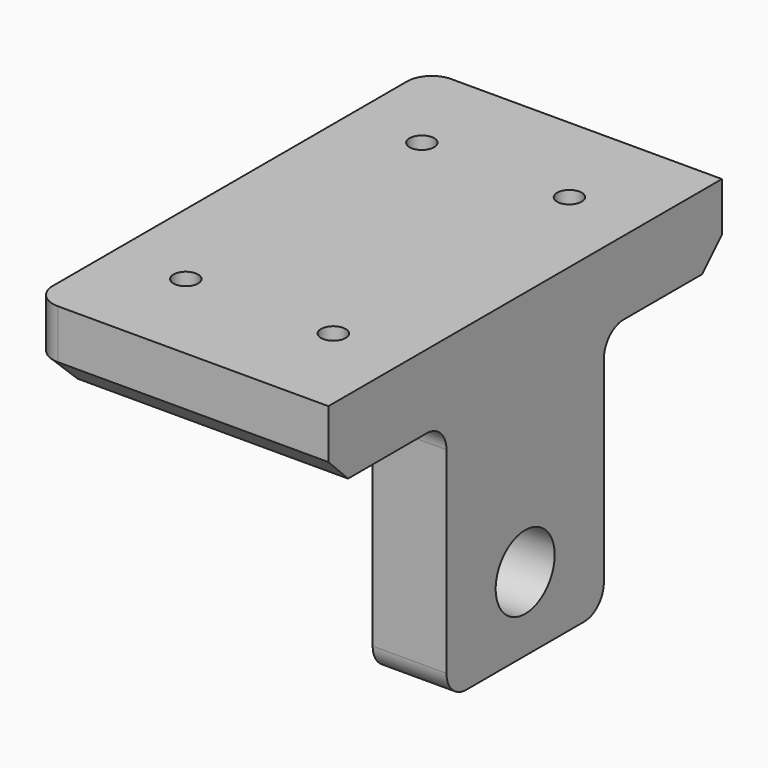
from build123d import *

# Parameters (mm, degrees)
F1_DEPTH  = 15
F2_W      = 40
F2_H      = 50
F3_DEPTH  = 15
F5_R      = 5
F6_SIZE   = 4.99999
F8_DEPTH  = 25
F9_R      = 2.5
F10_DEPTH = 25


# Not quite as in the source:
# - a fillet or chamfer is up to 0.001 mm smaller than in the source, because OpenCascade refuses the exact size


with BuildPart() as f1:
    # F0 (on Top) → F1 (new body)
    with BuildSketch(Plane.XY):
        with BuildLine():
            Line((30, 50), (-25, 50))
            ThreePointArc((-25, 50), (-28.5355339059, 48.5355339059), (-30, 45))
            Line((-30, 45), (-30, -45))
            ThreePointArc((-30, -45), (-28.5355339059, -48.5355339059), (-25, -50))
            Line((-25, -50), (30, -50))
            Line((30, -50), (30, 50))
        make_face()
    extrude(amount=F1_DEPTH)


with BuildPart() as f3:
    # F2 (on face) → F3 (new body)
    with BuildSketch(Plane.YZ.offset(30)):
        with Locations((0, -25)):
            Rectangle(F2_W, F2_H)
    extrude(amount=-F3_DEPTH)

    # F4: union F1
    add(f1.part)

    # F5
    f5_edges = [f3.edges().sort_by_distance(p)[0] for p in [
        (15, 0, 0),
        (22.5, 20, -50),
        (22.5, -20, -50),
        (22.5, 20, 0),
        (22.5, -20, 0),
    ]]
    fillet(f5_edges, radius=F5_R)

    # F6 (size 5 in the source; OpenCascade refuses exactly that, so slightly less here)
    f6_edges = [f3.edges().sort_by_distance(p)[0] for p in [
        (-30, 0, 0),
        (2.5, 50, 0),
        (2.5, -50, 0),
    ]]
    chamfer(f6_edges, length=F6_SIZE)

    # F7 (on face) → F8 (cut)
    with BuildSketch(Plane(origin=(15, 0, 0), x_dir=(0, -1, 0), z_dir=(-1, 0, 0))):
        with BuildLine():
            Line((0, -27.5), (0, -42.5))
            ThreePointArc((0, -42.5), (5.3033008589, -40.3033008589), (7.5, -35))
            ThreePointArc((7.5, -35), (5.3033008589, -29.6966991411), (0, -27.5))
        make_face()
        with BuildLine():
            ThreePointArc((0, -27.5), (-7.5, -35), (0, -42.5))
            Line((0, -42.5), (0, -27.5))
        make_face()
    extrude(amount=-F8_DEPTH, mode=Mode.SUBTRACT)

    # F9 (on face) → F10 (cut)
    with BuildSketch(Plane.XY.offset(15)):
        with Locations((-15, -30)):
            Circle(F9_R)
        with Locations((-15, 30)):
            Circle(F9_R)
        with Locations((15, -30)):
            Circle(F9_R)
        with Locations((15, 30)):
            Circle(F9_R)
    extrude(amount=-F10_DEPTH, mode=Mode.SUBTRACT)


solid = f3.part
